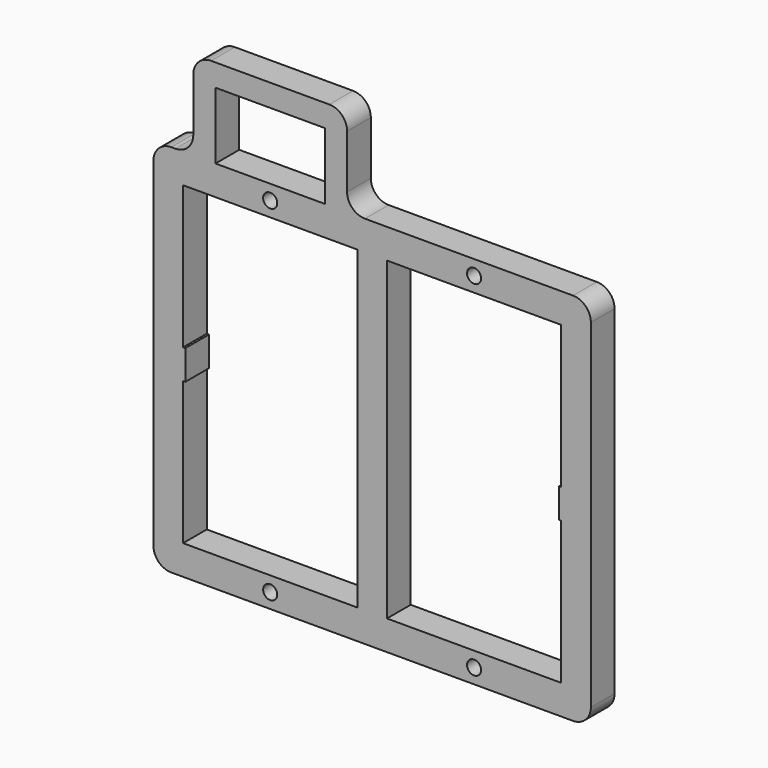
from build123d import *

# Parameters (mm, degrees)
F0_W     = 14.75
F0_H     = 9
F1_DEPTH = 4
F2_R     = 2.4
F3_D     = 1.9


with BuildPart() as f1:
    # F0 (on Front) → F1 (new body)
    with BuildSketch(Plane.XZ):
        Polygon((-24.125, 46.5), (-29.5, 46.5), (-29.5, -4), (29.5, -4), (29.5, 46.5), (-3.375, 46.5), (-3.375, 58.5), (-24.125, 58.5), align=None)
        Polygon((-2, 42.5), (-2, 0), (-25.5, 0), (-25.5, 19.25), (-25.2, 19.25), (-25.2, 23.25), (-25.5, 23.25), (-25.5, 42.5), align=None, mode=Mode.SUBTRACT)
        Polygon((25.5, 0), (2, 0), (2, 42.5), (25.5, 42.5), (25.5, 23.25), (25.2, 23.25), (25.2, 19.25), (25.5, 19.25), align=None, mode=Mode.SUBTRACT)
        with Locations((-13.75, 51)):
            Rectangle(F0_W, F0_H, mode=Mode.SUBTRACT)
    extrude(amount=F1_DEPTH)

    # F2
    f2_edges = [f1.edges().sort_by_distance(p)[0] for p in [
        (-24.125, -2, 58.5),
        (-24.125, -2, 46.5),
        (-29.5, -2, 46.5),
        (-3.375, -2, 58.5),
        (29.5, -2, 46.5),
        (-3.375, -2, 46.5),
        (29.5, -2, -4),
        (-29.5, -2, -4),
    ]]
    fillet(f2_edges, radius=F2_R)

    # F3 (through all)
    with Locations(Plane(origin=(0, 0, 0), x_dir=(1, 0, 0), z_dir=(0, 1, 0))):
        with Locations((-13.75, 2), (13.75, 2), (-13.75, -44.5), (13.75, -44.5)):
            Hole(F3_D / 2)


solid = f1.part
